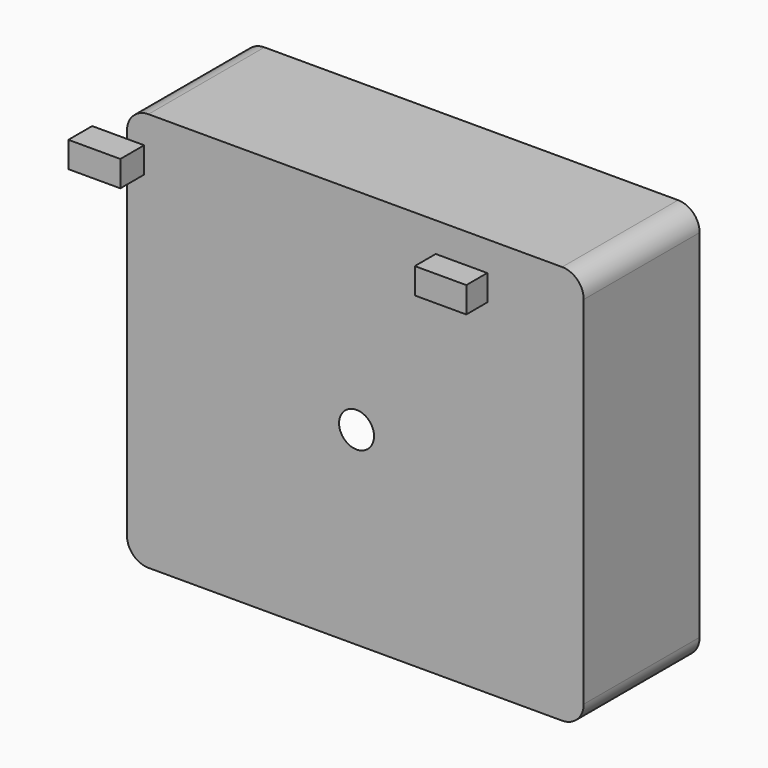
from build123d import *

# Parameters (mm, degrees)
F0_W        = 105.944249779
F0_H        = 92.6303975284
F1_DEPTH    = 33.6
F3_D        = 80
F3_DEPTH    = 12
F3_TIP      = 24.0344247611
F4_T1_DEPTH = 58.6
F5_W        = 12.0511576533
F5_H        = 6.9010909647
F6_DEPTH    = 6
F5_W_2      = 11.9481608272
F5_H_2      = 6.0770791024


# Not quite as in the source:
# - a fillet or chamfer that OpenCascade refuses, or shapes differently, is made with other operations: its cross-section is extruded or revolved along the edge and cut away or added


with BuildPart() as f1:
    # F0 (on Front) → F1 (new body)
    with BuildSketch(Plane.XZ):
        with Locations((-0.2832729369, 2.4078246206)):
            Rectangle(F0_W, F0_H)
    extrude(amount=-F1_DEPTH)

    # F3
    with Locations(Plane(origin=(0, 33.6, 0), x_dir=(-1, 0, 0), z_dir=(0, 1, 0))):
        with Locations((0, 0)):
            Hole(F3_D / 2, depth=F3_DEPTH)
            with Locations((0, 0, -(F3_DEPTH + F3_TIP / 2))):  # 118° drill point
                Cone(0, F3_D / 2, F3_TIP, mode=Mode.SUBTRACT)

    # F4: fillet of radius 5 on 5 edges, made by hand

    # F4_s2 → F4_t1 (cut)
    with BuildSketch(Plane.XZ.offset(-46.1)):
        with BuildLine():
            ThreePointArc((47.6888519526, 48.7230233848), (51.2243858585, 47.2585572907), (52.6888519526, 43.7230233848))
            Line((52.6888519526, 43.7230233848), (52.6888519526, 48.7230233848))
            Line((52.6888519526, 48.7230233848), (47.6888519526, 48.7230233848))
        make_face()
        with BuildLine():
            ThreePointArc((-48.2553978264, 48.7230233848), (-51.7909317324, 47.2585572907), (-53.2553978264, 43.7230233848))
            Line((-53.2553978264, 43.7230233848), (-53.2553978264, 48.7230233848))
            Line((-53.2553978264, 48.7230233848), (-48.2553978264, 48.7230233848))
        make_face()
        with BuildLine():
            ThreePointArc((-53.2553978264, -38.9073741436), (-51.7909317324, -42.4429080495), (-48.2553978264, -43.9073741436))
            Line((-48.2553978264, -43.9073741436), (-53.2553978264, -43.9073741436))
            Line((-53.2553978264, -43.9073741436), (-53.2553978264, -38.9073741436))
        make_face()
        with BuildLine():
            ThreePointArc((52.6888519526, -38.9073741436), (51.2243858585, -42.4429080495), (47.6888519526, -43.9073741436))
            Line((47.6888519526, -43.9073741436), (52.6888519526, -43.9073741436))
            Line((52.6888519526, -43.9073741436), (52.6888519526, -38.9073741436))
        make_face()
    extrude(amount=F4_T1_DEPTH, mode=Mode.SUBTRACT)

    # F4_s3 → F4_t4 (revolve, cut)
    with BuildSketch(Plane.XY):
        with BuildLine():
            ThreePointArc((-45, 33.6), (-41.4644660941, 32.1355339059), (-40, 28.6))
            Line((-40, 28.6), (-40, 33.6))
            Line((-40, 33.6), (-45, 33.6))
        make_face()
    revolve(axis=Axis((0, 33.6, 0), (0, 1, 0)), mode=Mode.SUBTRACT)


with BuildPart() as f6:
    # F5 (on face) → F6 (new body)
    with BuildSketch(Plane.XY.offset(48.7230233848)):
        with Locations((-40.0932952762, -22.448499687)):
            Rectangle(F5_W, F5_H)
    extrude(amount=F6_DEPTH)


with BuildPart() as f6b:
    # F5 (on face) → F6, piece 2 (new body)
    with BuildSketch(Plane.XY.offset(48.7230233848)):
        with Locations((39.7842526436, -22.3454991356)):
            Rectangle(F5_W_2, F5_H_2)
    extrude(amount=F6_DEPTH)


solid = Compound([f1.part, f6.part, f6b.part])
